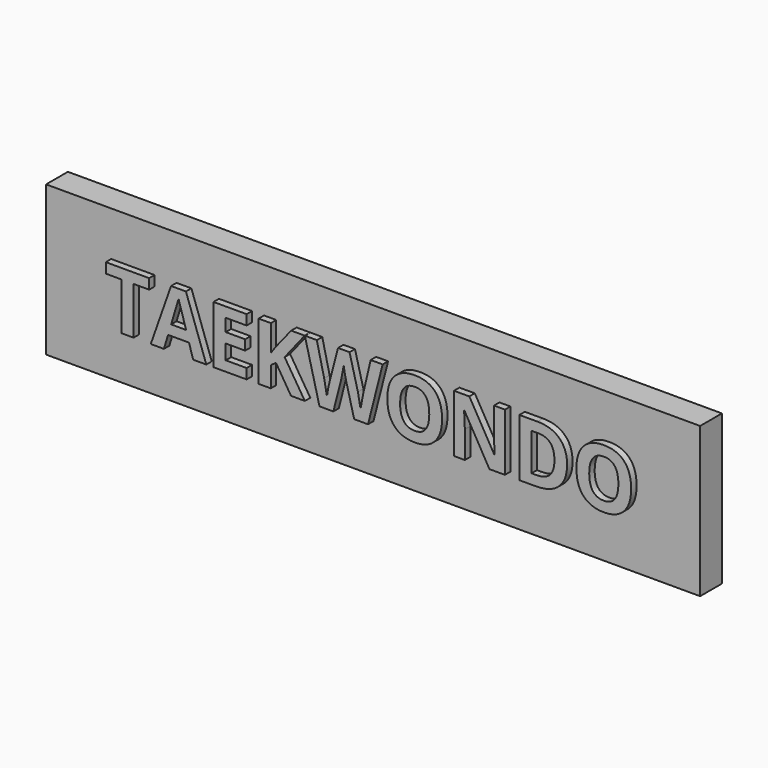
from build123d import *

# Parameters (mm, degrees)
F0_W         = 609.6
F0_H         = 25.4
F1_DEPTH     = 139.7
F2_TEXT_SIZE = 75.0249199983
F3_DEPTH     = 6.35


# Not quite as in the source:
# - Text() gives the source's letters only with a copy of the font that has no kerning and outlines rounded to 1/6400 em; it was checked with that copy


with BuildPart() as f1:
    # F0 (on Top) → F1 (new body)
    with BuildSketch(Plane.XY):
        with Locations((-304.8, 12.7)):
            Rectangle(F0_W, F0_H)
    extrude(amount=F1_DEPTH)

    # F2 (on face) → F3 (join)
    with BuildSketch(Plane.XZ):
        with Locations((-550.3952478789, 44.6505211294)):
            Text('TAEKWONDO', F2_TEXT_SIZE, font='Open Sans', font_style=FontStyle.BOLD, text_align=(TextAlign.LEFT, TextAlign.BOTTOM))
    extrude(amount=F3_DEPTH)


solid = f1.part
